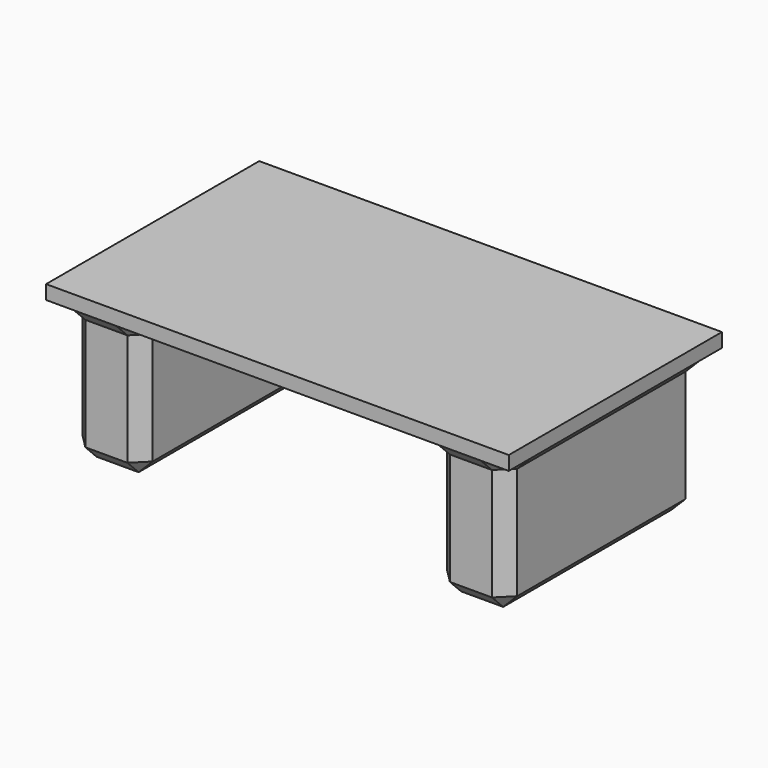
from build123d import *

# Parameters (mm, degrees)
F1_W     = 6.6
F1_H     = 3.8
F1_W_2   = 1
F1_H_2   = 3.4
F3_DEPTH = 0.2
F4_DEPTH = 2
F5_SIZE  = 0.19999


# Not quite as in the source:
# - a fillet or chamfer is up to 0.001 mm smaller than in the source, because OpenCascade refuses the exact size
# - a feature names something its author has since deleted; it is built from what else it names


with BuildPart() as f3:
    # F1 (on Top) → F3 (new body)
    with BuildSketch(Plane.XY):
        with Locations((0, -0.0311205854)):
            Rectangle(F1_W, F1_H)
        with Locations((-2.6, -0.0311205854)):
            Rectangle(F1_W_2, F1_H_2, mode=Mode.SUBTRACT)
        with Locations((2.6, -0.0311205854)):
            Rectangle(F1_W_2, F1_H_2, mode=Mode.SUBTRACT)
        with Locations((-2.6, -0.0311205854)):
            Rectangle(F1_W_2, F1_H_2)
        with Locations((2.6, -0.0311205854)):
            Rectangle(F1_W_2, F1_H_2)
    extrude(amount=F3_DEPTH)

    # F1 (on Top) → F4 (join, through all)
    with BuildSketch(Plane.XY):
        with Locations((-2.6, -0.0311205854)):
            Rectangle(F1_W_2, F1_H_2)
        with Locations((2.6, -0.0311205854)):
            Rectangle(F1_W_2, F1_H_2)
    extrude(amount=-F4_DEPTH)

    # F5 (size 0.2 in the source; OpenCascade refuses exactly that, so slightly less here)
    f5_edges = [f3.edges().sort_by_distance(p)[0] for p in [
        (-3.1, -1.731121, -1),
        (-2.1, -1.731121, -1),
        (-2.6, -1.731121, 0),
        (-2.6, -1.731121, -2),
        (-3.1, 1.668879, -1),
        (-3.1, -0.031121, 0),
        (-3.1, -0.031121, -2),
        (-2.1, 1.668879, -1),
        (-2.1, -0.031121, 0),
        (-2.1, -0.031121, -2),
        (-2.6, 1.668879, 0),
        (-2.6, 1.668879, -2),
        (3.1, -1.731121, -1),
        (3.1, 1.668879, -1),
        (3.1, -0.031121, 0),
        (3.1, -0.031121, -2),
        (2.1, 1.668879, -1),
        (2.1, -1.731121, -1),
        (2.1, -0.031121, 0),
        (2.1, -0.031121, -2),
        (2.6, -1.731121, 0),
        (2.6, -1.731121, -2),
        (2.6, 1.668879, 0),
        (2.6, 1.668879, -2),
    ]]
    chamfer(f5_edges, length=F5_SIZE)


solid = f3.part
